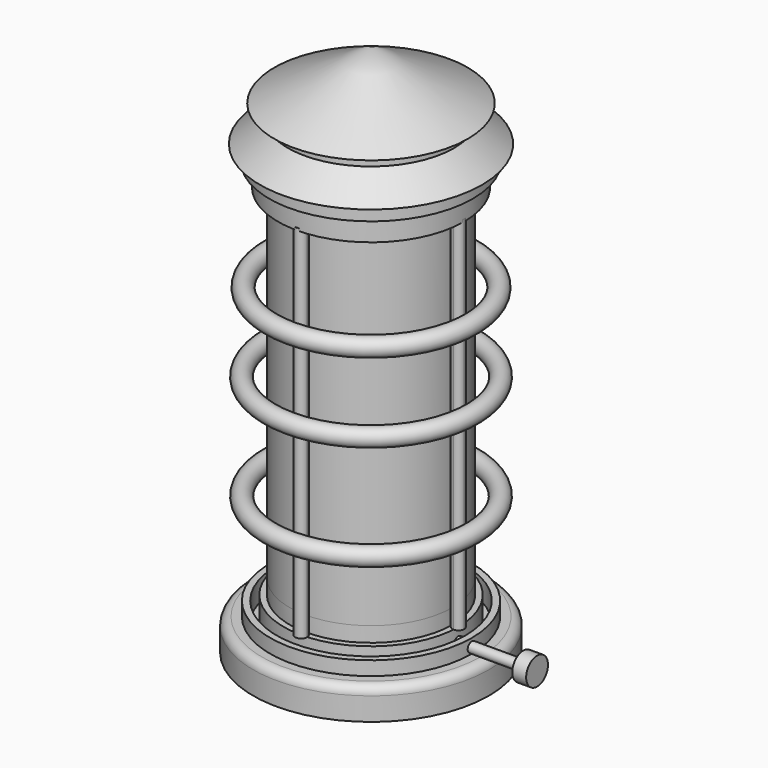
from build123d import *

# Parameters (mm, degrees)
F2_R      = 45.8683508663
F3_DEPTH  = 12.2300032526
F4_R      = 3.3243260017
F5_R      = 39.2446138712
F6_DEPTH  = 5.4330164567
F7_T      = -2.54
F8_R      = 33.9480342633
F9_DEPTH  = 17.1563792974
F10_R     = 31.6510256054
F11_DEPTH = 5.8644730598
F13_DEPTH = 140.4532641172
F14_DEPTH = 134.5577389002
F15_T     = -0.0254
F16_DEPTH = 133.6130052805
F17_R     = 36.1767908596
F18_DEPTH = 8.9578405023
F19_R     = 39.5916894085
F19_R_2   = 36.1767908596
F20_DEPTH = 6.1409324408
F23_R     = 5.3493148044
F24_DEPTH = 28.7772919983
F27_R     = 3.4354229328
F27_R_2   = 3.4924611579
F27_R_3   = 3.5031451318
F31_R     = 1.9898060625
F32_DEPTH = 64.5959377289
F33_R     = 5.3126821934
F33_R_2   = 1.9898060625
F34_DEPTH = 5.3814365529


# Not quite as in the source:
# - the program builds the solid bodies; features that only make, move or delete a surface that nothing else refers to are left out


with BuildPart() as f3:
    # F2 (on face) → F3 (new body)
    with BuildSketch(Plane.XY.offset(-40.9361049533)):
        Circle(F2_R)
    extrude(amount=F3_DEPTH)

    # F4
    f4_edges = [f3.edges().sort_by_distance(p)[0] for p in [
        (-45.868351, 0, -28.706102),
    ]]
    fillet(f4_edges, radius=F4_R)

    # F5 (on face) → F6 (join)
    with BuildSketch(Plane.XY.offset(-28.7061017007)):
        Circle(F5_R)
    extrude(amount=F6_DEPTH)

    # F7
    f7_openings = [f3.faces().sort_by_distance(p)[0] for p in [
        (0, 0, -23.273085),
    ]]
    offset(amount=F7_T, openings=f7_openings, kind=Kind.INTERSECTION)

    # F8 (on face) → F9 (join)
    with BuildSketch(Plane.XY.offset(-38.3961049533)):
        Circle(F8_R)
    extrude(amount=F9_DEPTH)

    # F10 (on face) → F11 (join)
    with BuildSketch(Plane.XY.offset(-21.2397256559)):
        Circle(F10_R)
    extrude(amount=F11_DEPTH)


with BuildPart() as f13:
    # F12 (on face) → F13 (new body)
    with BuildSketch(Plane.XY.offset(-21.2397256559)):
        with BuildLine():
            ThreePointArc((33.8703235962, -2.2956937572), (35.5445533987, -1.6514767406), (36.2450429212, 0))
            ThreePointArc((36.2450429212, 0), (35.5445533987, 1.6514767406), (33.8703235962, 2.2956937572))
            ThreePointArc((33.8703235962, 2.2956937572), (33.9286010343, 1.1485043289), (33.9480342633, 0))
            ThreePointArc((33.9480342633, 0), (33.9286010343, -1.1485043289), (33.8703235962, -2.2956937572))
        make_face()
        with BuildLine():
            ThreePointArc((33.9480342633, 0), (33.9286010343, 1.1485043289), (33.8703235962, 2.2956937572))
            ThreePointArc((33.8703235962, 2.2956937572), (32.2965575227, 1.5965191354), (31.6510256054, 0))
            ThreePointArc((31.6510256054, 0), (32.2965575227, -1.5965191354), (33.8703235962, -2.2956937572))
            ThreePointArc((33.8703235962, -2.2956937572), (33.9286010343, -1.1485043289), (33.9480342633, 0))
        make_face()
    extrude(amount=F13_DEPTH)


with BuildPart() as f13b:
    # F12 (on face) → F13, piece 2 (new body)
    with BuildSketch(Plane.XY.offset(-21.2397256559)):
        with BuildLine():
            ThreePointArc((-33.8703235962, -2.2956937572), (-32.2965575227, -1.5965191354), (-31.6510256054, 0))
            ThreePointArc((-31.6510256054, 0), (-32.2965575227, 1.5965191354), (-33.8703235962, 2.2956937572))
            ThreePointArc((-33.8703235962, 2.2956937572), (-33.9480342633, 0), (-33.8703235962, -2.2956937572))
        make_face()
        with BuildLine():
            ThreePointArc((-33.8703235962, -2.2956937572), (-33.9480342633, 0), (-33.8703235962, 2.2956937572))
            ThreePointArc((-33.8703235962, 2.2956937572), (-36.2450429212, 0), (-33.8703235962, -2.2956937572))
        make_face()
    extrude(amount=F13_DEPTH)


with BuildPart() as f13c:
    # F12 (on face) → F13, piece 3 (new body)
    with BuildSketch(Plane.XY.offset(-21.2397256559)):
        with BuildLine():
            ThreePointArc((1.28e-08, 31.6510256054), (1.59651914, 32.2965575272), (2.2956937572, 33.8703235962))
            ThreePointArc((2.2956937572, 33.8703235962), (0, 33.9480342633), (-2.2956937572, 33.8703235962))
            ThreePointArc((-2.2956937572, 33.8703235962), (-1.5965191308, 32.2965575182), (1.28e-08, 31.6510256054))
        make_face()
        with BuildLine():
            ThreePointArc((-2.2956937572, 33.8703235962), (0, 33.9480342633), (2.2956937572, 33.8703235962))
            ThreePointArc((2.2956937572, 33.8703235962), (2.2966799092, 33.909173368), (2.2970086579, 33.9480342633))
            ThreePointArc((2.2970086579, 33.9480342633), (-0.0388608953, 36.2447141725), (-2.2956937572, 33.8703235962))
        make_face()
    extrude(amount=F13_DEPTH)


with BuildPart() as f13d:
    # F12 (on face) → F13, piece 4 (new body)
    with BuildSketch(Plane.XY.offset(-21.2397256559)):
        with BuildLine():
            ThreePointArc((2.3426547832, -33.9480342633), (2.3423060388, -33.9076133033), (2.3412599093, -33.867204378))
            ThreePointArc((2.3412599093, -33.867204378), (0, -33.9480342633), (-2.3412599093, -33.867204378))
            ThreePointArc((-2.3412599093, -33.867204378), (-0.04042096, -36.2903403021), (2.3426547832, -33.9480342633))
        make_face()
        with BuildLine():
            ThreePointArc((-2.3412599093, -33.867204378), (0, -33.9480342633), (2.3412599093, -33.867204378))
            ThreePointArc((2.3412599093, -33.867204378), (1.7807921495, -32.4259269235), (0.4443457961, -31.6479063871))
            ThreePointArc((0.4443457961, -31.6479063871), (0, -31.6510256054), (-0.4443457961, -31.6479063871))
            ThreePointArc((-0.4443457961, -31.6479063871), (-1.7807921495, -32.4259269235), (-2.3412599093, -33.867204378))
        make_face()
    extrude(amount=F13_DEPTH)


with BuildPart() as f14:
    # F14 (new): a face of the model
    f14_faces = [f3.part.faces().sort_by_distance(p)[0] for p in [
        (0, 0, -15.3752525961),
    ]]
    extrude(f14_faces, amount=F14_DEPTH)

    # F15
    f15_openings = [f14.faces().sort_by_distance(p)[0] for p in [
        (0, 0, 119.182486),
    ]]
    offset(amount=F15_T, openings=f15_openings)

    # F16 (add): a face of the model
    f16_faces = [f14.faces().sort_by_distance(p)[0] for p in [
        (0, 0, -15.3498525961),
    ]]
    extrude(f16_faces, amount=F16_DEPTH)


with BuildPart() as f18:
    # F17 (on face) → F18 (new body)
    with BuildSketch(Plane.XY.offset(118.2631526844)):
        Circle(F17_R)
    extrude(amount=F18_DEPTH)

    # F19 (on face) → F20 (join)
    with BuildSketch(Plane.XY.offset(127.2209931866)):
        Circle(F19_R)
        Circle(F19_R_2, mode=Mode.SUBTRACT)
        Circle(F19_R_2)
    extrude(amount=F20_DEPTH)

    # F23 (on face) → F24 (join)
    with BuildSketch(Plane.XY.offset(133.3619256274)):
        Circle(F23_R)
    extrude(amount=F24_DEPTH)

    # F25 (on Front) → F26 (revolve)
    with BuildSketch(Plane.XZ):
        Polygon((0, 166.4425432682), (0, 148.0017155409), (0, 133.1499069929), (43.1951247156, 133.1499069929), (32.345879823, 142.2440111637), (32.345879823, 147.077023983), (37.6156680286, 147.077023983), align=None)
    revolve(axis=Axis((0, 0, 157.2221294045), (0, 0, -1)))


with BuildPart() as f29:
    # F27 (on Right) → F29 (revolve)
    with BuildSketch(Plane.YZ):
        with Locations((-39.3823459744, 53.4491688013)):
            Circle(F27_R)
    revolve(axis=Axis((0, 0, -15.3752525961), (0, 0, -1)))


with BuildPart() as f29b:
    # F27 (on Right) → F29, piece 2 (revolve)
    with BuildSketch(Plane.YZ):
        with Locations((-39.3060073256, 12.6033835113)):
            Circle(F27_R_2)
    revolve(axis=Axis((0, 0, -15.3752525961), (0, 0, -1)))


with BuildPart() as f29c:
    # F27 (on Right) → F29, piece 3 (revolve)
    with BuildSketch(Plane.YZ):
        with Locations((-38.8865955174, 84.078207612)):
            Circle(F27_R_3)
    revolve(axis=Axis((0, 0, -15.3752525961), (0, 0, -1)))


with BuildPart() as f30:
    # F27 (on Right) → F30 (revolve)
    with BuildSketch(Plane.YZ):
        with Locations((-39.3823459744, 53.4491688013)):
            Circle(F27_R)
    revolve(axis=Axis((0, 0, -15.3752525961), (0, 0, -1)))


with BuildPart() as f30b:
    # F27 (on Right) → F30, piece 2 (revolve)
    with BuildSketch(Plane.YZ):
        with Locations((-39.3060073256, 12.6033835113)):
            Circle(F27_R_2)
    revolve(axis=Axis((0, 0, -15.3752525961), (0, 0, -1)))


with BuildPart() as f30c:
    # F27 (on Right) → F30, piece 3 (revolve)
    with BuildSketch(Plane.YZ):
        with Locations((-38.8865955174, 84.078207612)):
            Circle(F27_R_3)
    revolve(axis=Axis((0, 0, -15.3752525961), (0, 0, -1)))


with BuildPart() as f3_1:
    add(f3.part)

    # F31 (on Right) → F32 (join)
    with BuildSketch(Plane.YZ):
        with Locations((0, -26.4002531767)):
            Circle(F31_R)
    extrude(amount=F32_DEPTH)

    # F33 (on face) → F34 (join)
    with BuildSketch(Plane.YZ.offset(64.5959377289)):
        with Locations((0, -26.4002531767)):
            Circle(F33_R)
        with Locations((0, -26.4002531767)):
            Circle(F33_R_2, mode=Mode.SUBTRACT)
        with Locations((0, -26.4002531767)):
            Circle(F33_R_2)
    extrude(amount=-F34_DEPTH)


solid = Compound([f13.part, f13b.part, f13c.part, f13d.part, f14.part, f18.part, f29.part, f29b.part, f29c.part, f30.part, f30b.part, f30c.part, f3_1.part])
